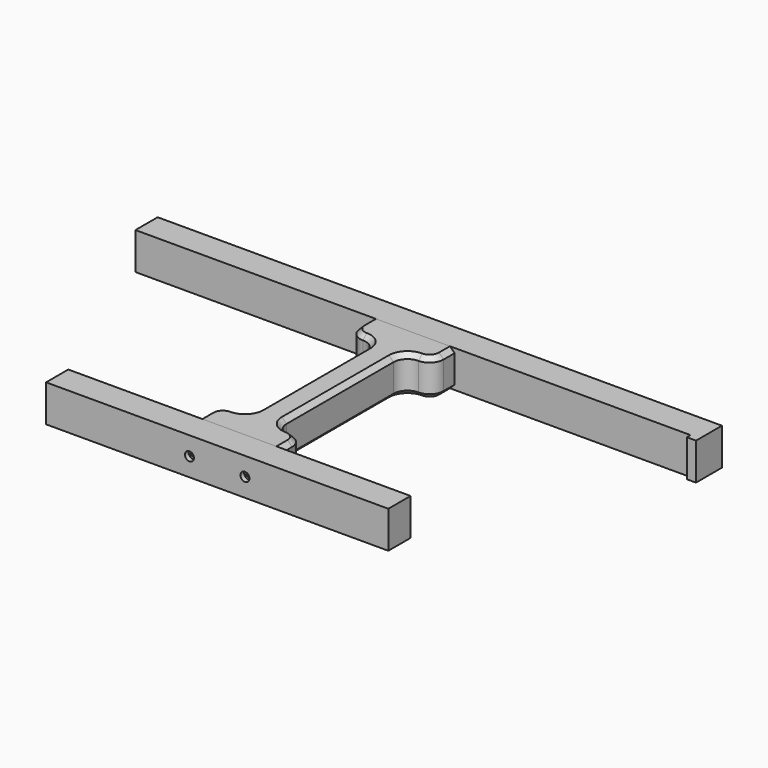
from build123d import *

# Parameters (mm, degrees)
F1_DEPTH             = 40
F0_W                 = 30
F0_H                 = 30
F2_DEPTH             = 40
F3_DEPTH             = 40
F4_R                 = 14.99999
F5_SIZE              = 5
F8_D                 = 5.3
F8_CBORE_D           = 9.75
F8_CBORE_DEPTH       = 5
F8_2_D               = 5.3
F8_2_CBORE_D         = 9.75
F8_2_CBORE_DEPTH     = 5
F8_ON_F7_D           = 5.3
F8_ON_F7_CBORE_D     = 9.75
F8_ON_F7_CBORE_DEPTH = 5
F9_D                 = 4.2
F9_DEPTH             = 17.4
F9_START             = 30
F9_TIP               = 1.2618073
F9_ON_F7_D           = 4.2
F9_ON_F7_DEPTH       = 17.4
F9_ON_F7_START       = 30
F9_ON_F7_TIP         = 1.2618073


# Not quite as in the source:
# - a fillet or chamfer is up to 0.001 mm smaller than in the source, because OpenCascade refuses the exact size


with BuildPart() as f1:
    # F0 (on Top) → F1 (new body)
    with BuildSketch(Plane.XY):
        Polygon((300, 294.5), (-300, 294.5), (-300, 264.5), (-45, 264.5), (-15, 264.5), (15, 264.5), (45, 264.5), (300, 264.5), align=None)
        Polygon((310, 294.5), (300, 294.5), (300, 264.5), (300, 259.5), (310, 259.5), align=None)
    extrude(amount=F1_DEPTH)

    # F8 (through all)
    with Locations(Plane(origin=(0, 294.5, 0), x_dir=(-1, 0, 0), z_dir=(0, 1, 0))):
        with Locations((-30, 20), (30, 20)):
            CounterBoreHole(F8_D / 2, F8_CBORE_D / 2, F8_CBORE_DEPTH)


with BuildPart() as f2:
    # F0 (on Top) → F2 (new body)
    with BuildSketch(Plane.XY):
        Polygon((15, 264.5), (-15, 264.5), (-15, 234.5), (-15, 60), (-15, 30), (15, 30), (15, 60), (15, 234.5), align=None)
        with Locations((-30, 249.5)):
            Rectangle(F0_W, F0_H)
        with Locations((30, 249.5)):
            Rectangle(F0_W, F0_H)
        with Locations((-30, 45)):
            Rectangle(F0_W, F0_H)
        with Locations((30, 45)):
            Rectangle(F0_W, F0_H)
    extrude(amount=F2_DEPTH)

    # F4 (radius 15 in the source; OpenCascade refuses exactly that, so slightly less here)
    f4_edges = [f2.edges().sort_by_distance(p)[0] for p in [
        (45, 234.5, 20),
        (-45, 234.5, 20),
        (-45, 60, 20),
        (45, 60, 20),
        (15, 234.5, 20),
        (-15, 234.5, 20),
        (-15, 60, 20),
        (15, 60, 20),
    ]]
    fillet(f4_edges, radius=F4_R)

    # F5
    f5_edges = [f2.edges().sort_by_distance(p)[0] for p in [
        (-15, 147.25, 40),
        (15, 147.25, 40),
        (-15, 147.25, 0),
        (15, 147.25, 0),
    ]]
    chamfer(f5_edges, length=F5_SIZE)

    # F9
    # its depths count from where the whole tool has entered the part; down to there all is cleared
    with Locations(Plane(origin=(0, 294.5, 0), x_dir=(-1, 0, 0), z_dir=(0, 1, 0))):
        with Locations((30, 20), (-30, 20)):
            Hole(F9_D / 2, depth=F9_START)
    with Locations(Plane(origin=(0, 294.5, 0), x_dir=(-1, 0, 0), z_dir=(0, 1, 0)).offset(-F9_START)):
        with Locations((30, 20), (-30, 20)):
            Hole(F9_D / 2, depth=F9_DEPTH)
            with Locations((0, 0, -(F9_DEPTH + F9_TIP / 2))):  # 118° drill point
                Cone(0, F9_D / 2, F9_TIP, mode=Mode.SUBTRACT)

    # F9 on F7
    # its depths count from where the whole tool has entered the part; down to there all is cleared
    with Locations(Plane.XZ):
        with Locations((-30, 20), (30, 20)):
            Hole(F9_ON_F7_D / 2, depth=F9_ON_F7_START)
    with Locations(Plane.XZ.offset(-F9_ON_F7_START)):
        with Locations((-30, 20), (30, 20)):
            Hole(F9_ON_F7_D / 2, depth=F9_ON_F7_DEPTH)
            with Locations((0, 0, -(F9_ON_F7_DEPTH + F9_ON_F7_TIP / 2))):  # 118° drill point
                Cone(0, F9_ON_F7_D / 2, F9_ON_F7_TIP, mode=Mode.SUBTRACT)


with BuildPart() as f3:
    # F0 (on Top) → F3 (new body)
    with BuildSketch(Plane.XY):
        Polygon((15, 30), (-15, 30), (-45, 30), (-185, 30), (-185, 0), (185, 0), (185, 30), (45, 30), align=None)
    extrude(amount=F3_DEPTH)

    # F8#2 (through all)
    with Locations(Plane(origin=(0, 294.5, 0), x_dir=(-1, 0, 0), z_dir=(0, 1, 0))):
        with Locations((-30, 20), (30, 20)):
            CounterBoreHole(F8_2_D / 2, F8_2_CBORE_D / 2, F8_2_CBORE_DEPTH)

    # F8 on F7 (through all)
    with Locations(Plane.XZ):
        with Locations((-30, 20), (30, 20)):
            CounterBoreHole(F8_ON_F7_D / 2, F8_ON_F7_CBORE_D / 2, F8_ON_F7_CBORE_DEPTH)


solid = Compound([f1.part, f2.part, f3.part])
